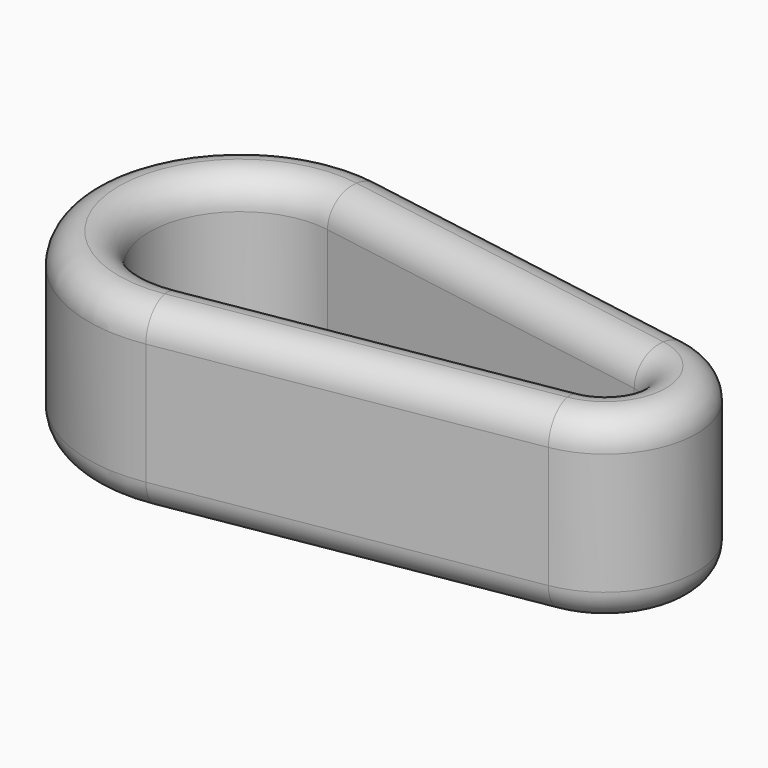
from build123d import *

# Parameters (mm, degrees)
F1_DEPTH = 30
F2_R     = 4.99999


# Not quite as in the source:
# - a fillet or chamfer is up to 0.001 mm smaller than in the source, because OpenCascade refuses the exact size


with BuildPart() as f1:
    # F0 (on Top) → F1 (new body)
    with BuildSketch(Plane.XY):
        with BuildLine():
            Line((62.5, 14.7901994577), (4.1666666667, 24.6503324296))
            ThreePointArc((4.1666666667, 24.6503324296), (-25, 0), (4.1666666667, -24.6503324296))
            Line((4.1666666667, -24.6503324296), (62.5, -14.7901994577))
            ThreePointArc((62.5, -14.7901994577), (75, 0), (62.5, 14.7901994577))
        make_face()
        with BuildLine():
            Line((60.8333333333, -4.9300664859), (2.5, -14.7901994577))
            ThreePointArc((2.5, -14.7901994577), (-15, 0), (2.5, 14.7901994577))
            Line((2.5, 14.7901994577), (60.8333333333, 4.9300664859))
            ThreePointArc((60.8333333333, 4.9300664859), (65, 0), (60.8333333333, -4.9300664859))
        make_face(mode=Mode.SUBTRACT)
    extrude(amount=F1_DEPTH)

    # F2 (radius 5 in the source; OpenCascade refuses exactly that, so slightly less here)
    f2_edges = [f1.edges().sort_by_distance(p)[0] for p in [
        (33.333333, -19.720266, 30),
        (75, 0, 30),
        (33.333333, 19.720266, 30),
        (-25, 0, 30),
        (31.666667, -9.860133, 30),
        (-15, 0, 30),
        (31.666667, 9.860133, 30),
        (65, 0, 30),
        (33.333333, -19.720266, 0),
        (75, 0, 0),
        (33.333333, 19.720266, 0),
        (-25, 0, 0),
        (31.666667, -9.860133, 0),
        (-15, 0, 0),
        (31.666667, 9.860133, 0),
        (65, 0, 0),
    ]]
    fillet(f2_edges, radius=F2_R)


solid = f1.part
